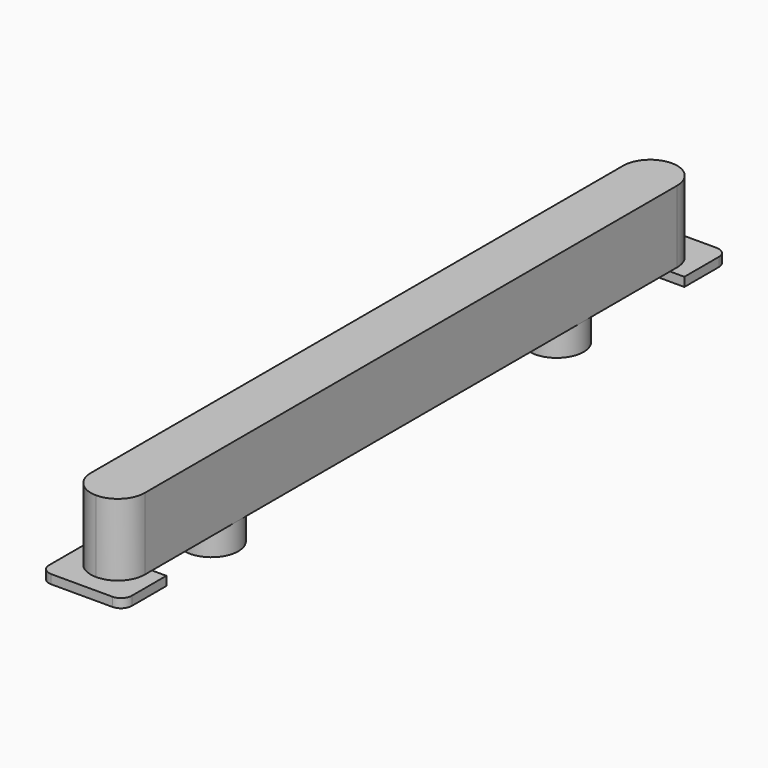
from build123d import *

# Parameters (mm, degrees)
F0_W     = 1.5
F0_H     = 1
F1_DEPTH = 2
F2_DEPTH = 0.25
F3_DEPTH = 0.75
F4_R     = 0.74999
F5_R     = 0.3


# Not quite as in the source:
# - a fillet or chamfer is up to 0.001 mm smaller than in the source, because OpenCascade refuses the exact size


with BuildPart() as f1:
    # F0 (on Top) → F1 (new body)
    with BuildSketch(Plane.XY):
        with Locations((-0.75, 9.1787409857)):
            Rectangle(F0_W, F0_H)
        with BuildLine():
            Line((0, 8.6787409857), (-1.5, 8.6787409857))
            Line((-1.5, 8.6787409857), (-1.5, 5.6787409857))
            ThreePointArc((-1.5, 5.6787409857), (-0.75, 6.4287409857), (0, 5.6787409857))
            Line((0, 5.6787409857), (0, 8.6787409857))
        make_face()
        with BuildLine():
            ThreePointArc((0, 5.6787409857), (-0.75, 6.4287409857), (-1.5, 5.6787409857))
            ThreePointArc((-1.5, 5.6787409857), (-0.75, 4.9287409857), (0, 5.6787409857))
        make_face()
        with BuildLine():
            ThreePointArc((0, 5.6787409857), (-0.75, 4.9287409857), (-1.5, 5.6787409857))
            Line((-1.5, 5.6787409857), (-1.5, -6.3212590143))
            ThreePointArc((-1.5, -6.3212590143), (-0.75, -5.5712590143), (0, -6.3212590143))
            Line((0, -6.3212590143), (0, 5.6787409857))
        make_face()
        with BuildLine():
            ThreePointArc((0, -6.3212590143), (-0.75, -5.5712590143), (-1.5, -6.3212590143))
            ThreePointArc((-1.5, -6.3212590143), (-0.75, -7.0712590143), (0, -6.3212590143))
        make_face()
        with BuildLine():
            ThreePointArc((0, -6.3212590143), (-0.75, -7.0712590143), (-1.5, -6.3212590143))
            Line((-1.5, -6.3212590143), (-1.5, -9.3212590143))
            Line((-1.5, -9.3212590143), (0, -9.3212590143))
            Line((0, -9.3212590143), (0, -6.3212590143))
        make_face()
        with Locations((-0.75, -9.8212590143)):
            Rectangle(F0_W, F0_H)
    extrude(amount=F1_DEPTH)

    # F0 (on Top) → F2 (join)
    with BuildSketch(Plane.XY):
        with Locations((-0.75, -9.8212590143)):
            Rectangle(F0_W, F0_H)
        Polygon((-1.5, -10.3212590143), (-1.5, -9.3212590143), (-1.9, -9.3212590143), (-1.9, -10.8212590143), (0.4, -10.8212590143), (0.4, -9.3212590143), (0, -9.3212590143), (0, -10.3212590143), align=None)
        Polygon((-1.5, 8.6787409857), (-1.5, 9.6787409857), (0, 9.6787409857), (0, 8.6787409857), (0.4, 8.6787409857), (0.4, 10.1787409857), (-1.9, 10.1787409857), (-1.9, 8.6787409857), align=None)
        with Locations((-0.75, 9.1787409857)):
            Rectangle(F0_W, F0_H)
    extrude(amount=-F2_DEPTH)

    # F0 (on Top) → F3 (join)
    with BuildSketch(Plane.XY):
        with BuildLine():
            ThreePointArc((0, -6.3212590143), (-0.75, -5.5712590143), (-1.5, -6.3212590143))
            ThreePointArc((-1.5, -6.3212590143), (-0.75, -7.0712590143), (0, -6.3212590143))
        make_face()
        with BuildLine():
            ThreePointArc((0, 5.6787409857), (-0.75, 6.4287409857), (-1.5, 5.6787409857))
            ThreePointArc((-1.5, 5.6787409857), (-0.75, 4.9287409857), (0, 5.6787409857))
        make_face()
    extrude(amount=-F3_DEPTH)

    # F4 (radius 0.75 in the source; OpenCascade refuses exactly that, so slightly less here)
    f4_edges = [f1.edges().sort_by_distance(p)[0] for p in [
        (0, 9.678741, 1),
        (-1.5, 9.678741, 1),
        (0, -10.321259, 1),
        (-1.5, -10.321259, 1),
    ]]
    fillet(f4_edges, radius=F4_R)

    # F5
    f5_edges = [f1.edges().sort_by_distance(p)[0] for p in [
        (0.4, 10.178741, -0.125),
        (-1.9, 10.178741, -0.125),
        (0.4, -10.821259, -0.125),
        (-1.9, -10.821259, -0.125),
    ]]
    fillet(f5_edges, radius=F5_R)


solid = f1.part
